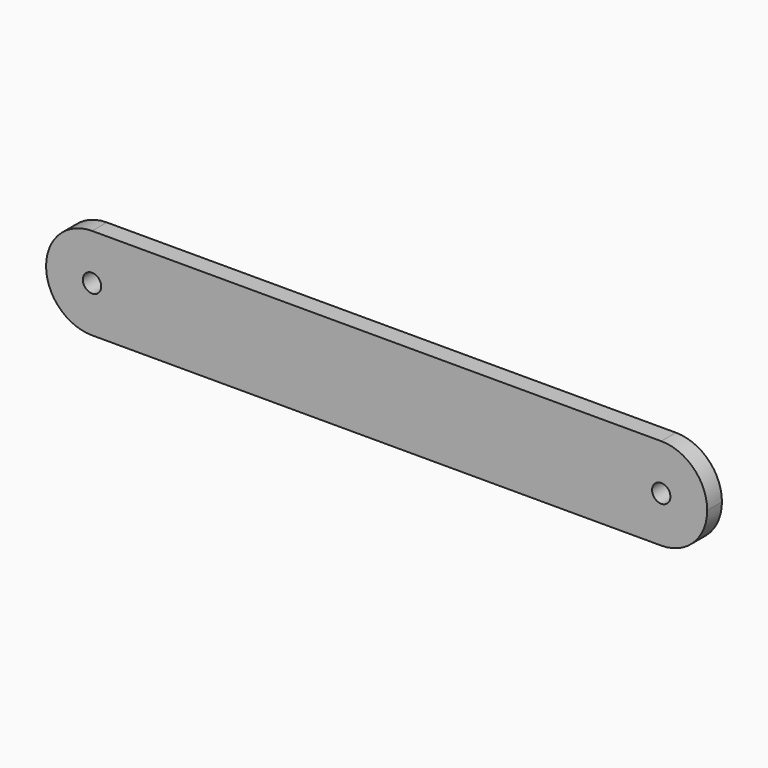
from build123d import *

# Parameters (mm, degrees)
F0_W     = 71.9
F0_H     = 10
F0_R     = 1
F1_DEPTH = 2
F2_R     = 4.99999


# Not quite as in the source:
# - a fillet or chamfer is up to 0.001 mm smaller than in the source, because OpenCascade refuses the exact size


with BuildPart() as f1:
    # F0 (on Front) → F1 (new body)
    with BuildSketch(Plane.XZ):
        with Locations((35.95, -5)):
            Rectangle(F0_W, F0_H)
        with Locations((5, -5)):
            Circle(F0_R, mode=Mode.SUBTRACT)
        with Locations((66.9, -5)):
            Circle(F0_R, mode=Mode.SUBTRACT)
    extrude(amount=F1_DEPTH)

    # F2 (radius 5 in the source; OpenCascade refuses exactly that, so slightly less here)
    f2_edges = [f1.edges().sort_by_distance(p)[0] for p in [
        (0, -1, 0),
        (0, -1, -10),
        (71.9, -1, 0),
        (71.9, -1, -10),
    ]]
    fillet(f2_edges, radius=F2_R)


solid = f1.part
